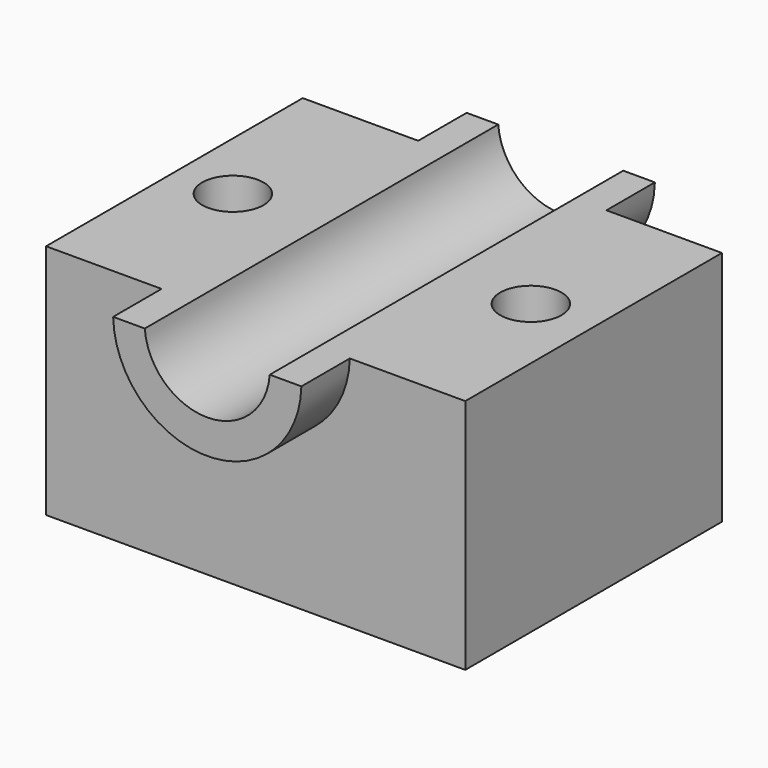
from build123d import *

# Parameters (mm, degrees)
F0_W          = 83.8607475162
F0_H          = 64.1791447997
F1_DEPTH      = 48.26
F2_R          = 18.8345255186
F3_DEPTH      = 44.196
F3_DEPTH_BACK = 44.196
F4_R          = 12.5378078108
F5_DEPTH      = 44.197
F5_DEPTH_BACK = 44.197
F7_DEPTH      = 44.197
F7_DEPTH_BACK = 44.197
F8_R          = 6.1393043091
F8_R_2        = 6.139306213
F9_DEPTH      = 154
F9_DEPTH_BACK = 47.3427378962


# Not quite as in the source:
# - an extrude ends at something that could not be found from the text; its depth is read off the source's solid


with BuildPart() as f1:
    # F0 (on Top) → F1 (new body)
    with BuildSketch(Plane.XY):
        Rectangle(F0_W, F0_H)
    extrude(amount=F1_DEPTH)

    # F2 (on Front) → F3 (join, two sides)
    with BuildSketch(Plane.XZ) as f3_sk:
        with Locations((0, 47.7778092027)):
            Circle(F2_R)
    extrude(amount=F3_DEPTH)
    extrude(f3_sk.sketch, amount=-F3_DEPTH_BACK)

    # F4 (on Front) → F5 (cut, two sides)
    with BuildSketch(Plane.XZ) as f5_sk:
        with Locations((0, 48.2809320092)):
            Circle(F4_R)
    extrude(amount=-F5_DEPTH, mode=Mode.SUBTRACT)
    extrude(f5_sk.sketch, amount=F5_DEPTH_BACK, mode=Mode.SUBTRACT)

    # F6 (on Front) → F7 (cut, two sides)
    with BuildSketch(Plane.XZ) as f7_sk:
        Polygon((-43.335814029, 47.3417378962), (42.9494790733, 47.3417378962), (48.3834594488, 70.2134892344), (-43.335814029, 70.2134892344), align=None)
    extrude(amount=-F7_DEPTH, mode=Mode.SUBTRACT)
    extrude(f7_sk.sketch, amount=F7_DEPTH_BACK, mode=Mode.SUBTRACT)

    # F8 (on Top) → F9 (cut, two sides)
    with BuildSketch(Plane.XY) as f9_sk:
        with Locations((-30.2355084568, 0)):
            Circle(F8_R)
        with Locations((29.3797850609, 0)):
            Circle(F8_R_2)
    extrude(amount=-F9_DEPTH, mode=Mode.SUBTRACT)
    extrude(f9_sk.sketch, amount=F9_DEPTH_BACK, mode=Mode.SUBTRACT)


solid = f1.part
